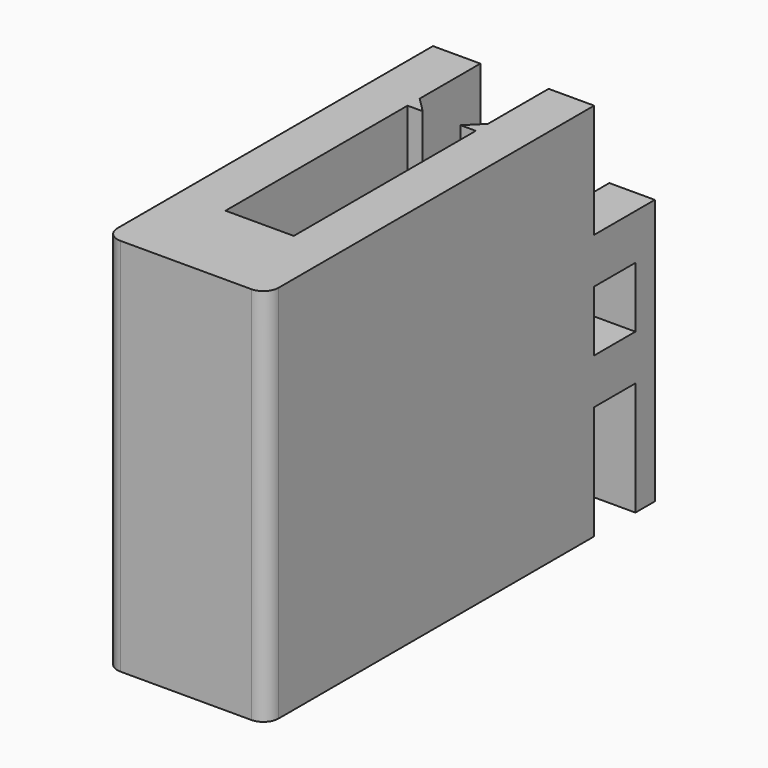
from build123d import *

# Parameters (mm, degrees)
F1_DEPTH = 25
F0_W     = 3.1244163401
F0_H     = 10
F0_W_2   = 3
F2_DEPTH = 25
F3_W     = 3.4
F3_H     = 4
F3_W_2   = 5
F3_H_2   = 7.5
F4_DEPTH = 25


# Not quite as in the source:
# - a feature names something its author has since deleted; it is built from what else it names


with BuildPart() as f1:
    # F0 (on Top) → F1 (new body)
    with BuildSketch(Plane.XY):
        with BuildLine():
            Line((4.5, 0), (0, 0))
            Line((0, 0), (0, 15))
            Line((0, 15), (1, 15))
            Line((1, 15), (0, 16))
            Line((0, 16), (-3.1244163401, 16))
            Line((-3.1244163401, 16), (-3.1244163401, 15))
            Line((-3.1244163401, 15), (-3.1244163401, 0))
            Line((-3.1244163401, 0), (-3.1244163401, -5))
            ThreePointArc((-3.1244163401, -5), (-2.8315231213, -5.7071067812), (-2.1244163401, -6))
            Line((-2.1244163401, -6), (4.5, -6))
            Line((4.5, -6), (6.5, -6))
            ThreePointArc((6.5, -6), (7.2071067812, -5.7071067812), (7.5, -5))
            Line((7.5, -5), (7.5, 15))
            Line((7.5, 15), (7.5, 16))
            Line((7.5, 16), (4.5, 16))
            Line((4.5, 16), (3.5, 15))
            Line((3.5, 15), (4.5, 15))
            Line((4.5, 15), (4.5, 0))
        make_face()
    extrude(amount=F1_DEPTH)

    # F0 (on Top) → F2 (join)
    with BuildSketch(Plane.XY):
        with BuildLine():
            Line((4.5, 0), (0, 0))
            Line((0, 0), (0, 15))
            Line((0, 15), (1, 15))
            Line((1, 15), (0, 16))
            Line((0, 16), (-3.1244163401, 16))
            Line((-3.1244163401, 16), (-3.1244163401, 15))
            Line((-3.1244163401, 15), (-3.1244163401, 0))
            Line((-3.1244163401, 0), (-3.1244163401, -5))
            ThreePointArc((-3.1244163401, -5), (-2.8315231213, -5.7071067812), (-2.1244163401, -6))
            Line((-2.1244163401, -6), (4.5, -6))
            Line((4.5, -6), (6.5, -6))
            ThreePointArc((6.5, -6), (7.2071067812, -5.7071067812), (7.5, -5))
            Line((7.5, -5), (7.5, 15))
            Line((7.5, 15), (7.5, 16))
            Line((7.5, 16), (4.5, 16))
            Line((4.5, 16), (3.5, 15))
            Line((3.5, 15), (4.5, 15))
            Line((4.5, 15), (4.5, 0))
        make_face()
        with Locations((-1.5622081701, 21)):
            Rectangle(F0_W, F0_H)
        with Locations((6, 21)):
            Rectangle(F0_W_2, F0_H)
    extrude(amount=F2_DEPTH)

    # F3 (on face) → F4 (cut)
    with BuildSketch(Plane.YZ.offset(7.5)):
        with Locations((22.7, 12.5)):
            Rectangle(F3_W, F3_H)
        with Locations((23.5, 21.25)):
            Rectangle(F3_W_2, F3_H_2)
        with Locations((22.7, 3.75)):
            Rectangle(F3_W, F3_H_2)
    extrude(amount=-F4_DEPTH, mode=Mode.SUBTRACT)


solid = f1.part
